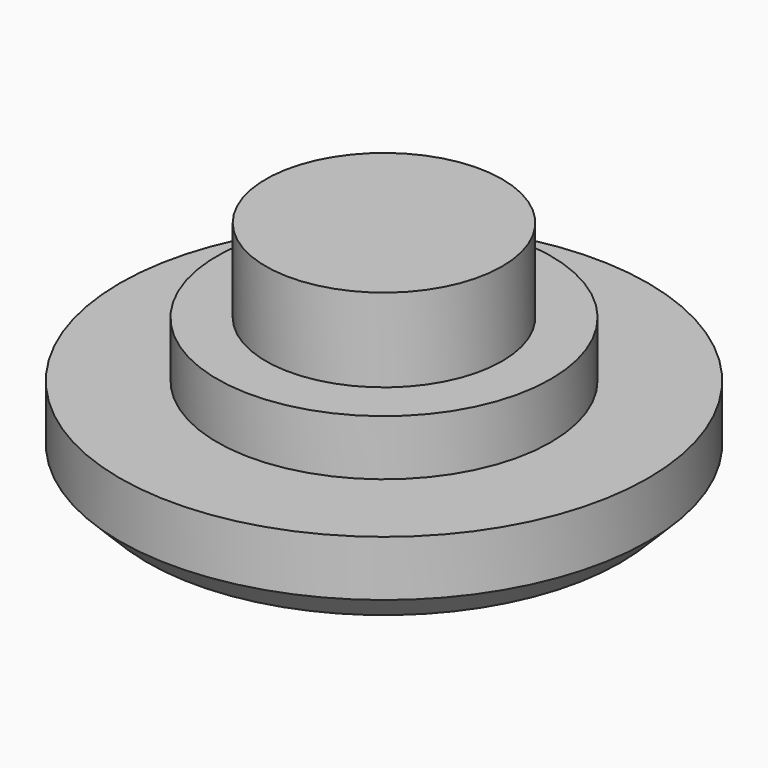
from build123d import *

# Parameters (mm, degrees)
F2_R         = 9.5
F2_R_2       = 6
F3_DEPTH     = 3
F2_R_3       = 4.25
F4_DEPTH     = 5
F5_DEPTH     = 8
F6_SIZE      = 1
F7_TEXT_SIZE = 18.6257230211
F8_DEPTH     = 1
F9_DEPTH     = 1


# Not quite as in the source:
# - Text() gives the source's letters only with a copy of the font that has no kerning and outlines rounded to 1/6400 em; it was checked with that copy


with BuildPart() as f3:
    # F2 (on Top) → F3 (new body)
    with BuildSketch(Plane.XY):
        Circle(F2_R)
        Circle(F2_R_2, mode=Mode.SUBTRACT)
    extrude(amount=F3_DEPTH)

    # F2 (on Top) → F4 (join)
    with BuildSketch(Plane.XY):
        Circle(F2_R_2)
        Circle(F2_R_3, mode=Mode.SUBTRACT)
    extrude(amount=F4_DEPTH)

    # F2 (on Top) → F5 (join)
    with BuildSketch(Plane.XY):
        Circle(F2_R_3)
    extrude(amount=F5_DEPTH)

    # F6
    f6_edges = [f3.edges().sort_by_distance(p)[0] for p in [
        (-9.5, 0, 0),
    ]]
    chamfer(f6_edges, length=F6_SIZE)

    # F7 (on face) → F8 (cut)
    with BuildSketch(Plane(origin=(0, 0, 0), x_dir=(1, 0, 0), z_dir=(0, 0, -1))):
        with Locations((-5.2258392485, -6.7067452099)):
            Text('L', F7_TEXT_SIZE, font='Open Sans', text_align=(TextAlign.LEFT, TextAlign.BOTTOM))
    extrude(amount=-F8_DEPTH, mode=Mode.SUBTRACT)

    # F7 (on face) → F9 (cut)
    with BuildSketch(Plane(origin=(0, 0, 0), x_dir=(1, 0, 0), z_dir=(0, 0, -1))):
        with Locations((-5.2258392485, -6.7067452099)):
            Text('L', F7_TEXT_SIZE, font='Open Sans', text_align=(TextAlign.LEFT, TextAlign.BOTTOM))
    extrude(amount=-F9_DEPTH, mode=Mode.SUBTRACT)


solid = f3.part
